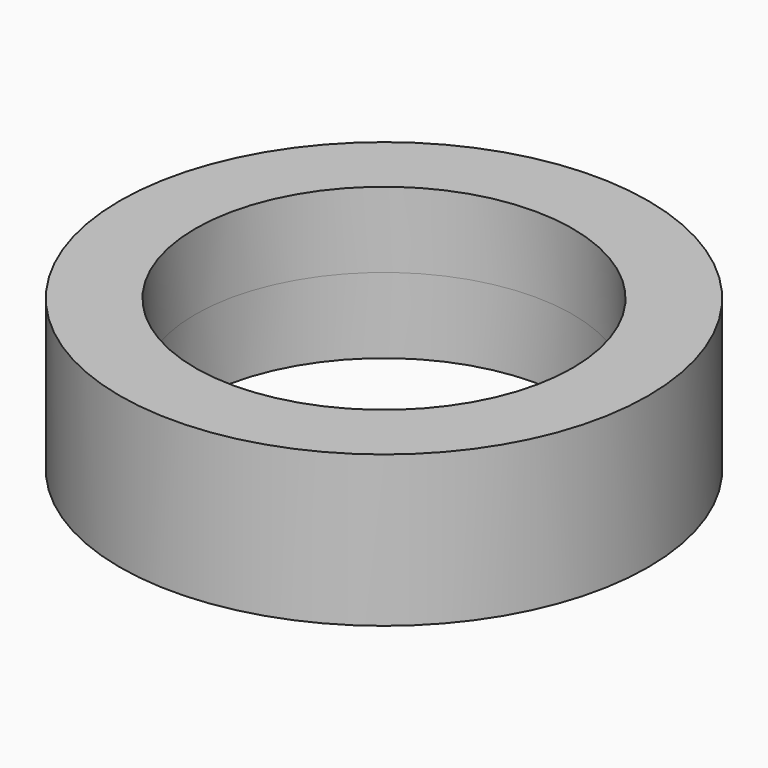
from build123d import *

# Parameters (mm, degrees)
F0_R     = 17.5
F0_R_2   = 12.5
F1_DEPTH = 5


# Not quite as in the source:
# - a feature of the source that left no trace in its solid (it failed there, or was rolled back) is left out
# - a pattern or mirror of a feature is missing from the dataset's text; its kind, count and spacing are read off the source's solid


with BuildPart() as f1:
    # F0 (on Top) → F1 (new body)
    with BuildSketch(Plane.XY):
        Circle(F0_R)
        Circle(F0_R_2, mode=Mode.SUBTRACT)
    extrude(amount=-F1_DEPTH)

    # F1_copies: F1 across plane


with BuildPart() as f1_1:
    add(f1.part)
    add(f1.part.mirror(Plane(origin=(0, 0, -5), x_dir=(-1, 0, 0), z_dir=(0, 0, -1))))


solid = f1_1.part
